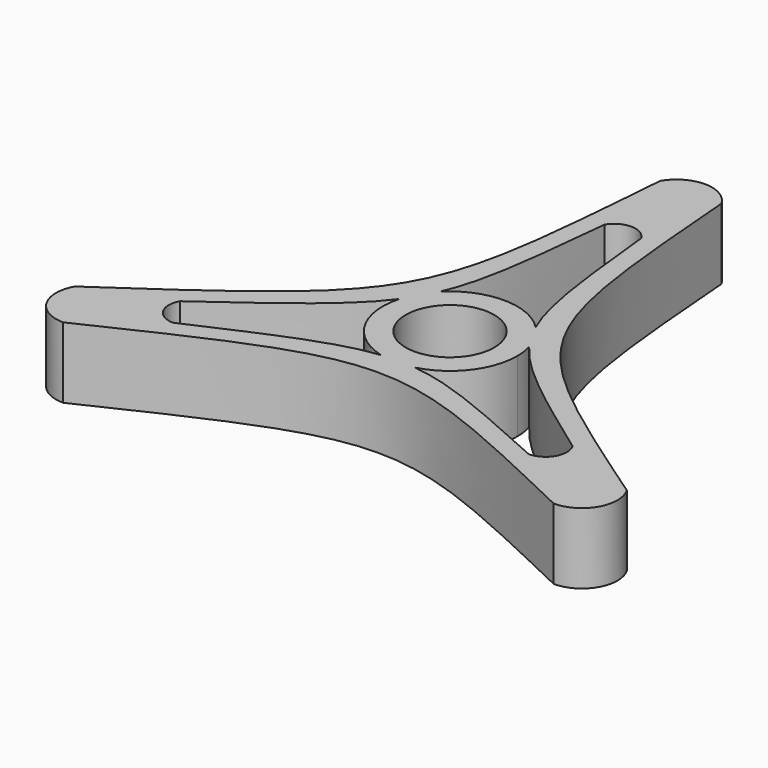
from build123d import *

# Parameters (mm, degrees)
F0_R     = 6.25
F1_DEPTH = 10


# Not quite as in the source:
# - a feature names something its author has since deleted; it is built from what else it names


with BuildPart() as f1:
    # F0 (on Top) → F1 (new body)
    with BuildSketch(Plane.XY):
        with BuildLine():
            add(Edge.make_bspline(
                [(4.3301272175, 42.4999999798), (7.3612159322, 4.25), (7.3612159322, 4.25), (38.9711430885, -17.5000001821)],
                knots=[0, 0, 0, 0, 69.2820323028, 69.2820323028, 69.2820323028, 69.2820323028], degree=3))
            ThreePointArc((4.3301272175, 42.4999999798), (2.102e-07, 45), (-4.3301268204, 42.5000000202))
            add(Edge.make_bspline(
                [(-38.9711432521, -17.4999998179), (-7.3612159322, 4.25), (-7.3612159322, 4.25), (-4.3301268204, 42.5000000202)],
                knots=[0, 0, 0, 0, 69.2820323028, 69.2820323028, 69.2820323028, 69.2820323028], degree=3))
            ThreePointArc((-38.9711432521, -17.4999998179), (-38.9711432754, -22.4999998179), (-34.6410162682, -24.9999998382))
            add(Edge.make_bspline(
                [(-34.6410162682, -24.9999998382), (0, -8.5), (0, -8.5), (34.6410160346, -25.0000001618)],
                knots=[0, 0, 0, 0, 69.2820323028, 69.2820323028, 69.2820323028, 69.2820323028], degree=3))
            ThreePointArc((34.6410160346, -25.0000001618), (38.9711430652, -22.5000001821), (38.9711430885, -17.5000001821))
        make_face()
        with BuildLine():
            ThreePointArc((6.7724364928, 6.6621395926), (8.2272413629, 4.7499999534), (9.1558004059, 2.5340321482))
            add(Edge.make_bspline(
                [(9.1558004059, 2.5340321482), (12.4794508791, -1.9849209314), (17.9661663578, -5.9523055453), (27.7128128343, -13.0000001849)],
                knots=[28.2758618531, 28.2758618531, 28.2758618531, 28.2758618531, 50.2294734195, 50.2294734195, 50.2294734195, 50.2294734195], degree=3))
            ThreePointArc((27.7128128343, -13.0000001849), (27.7128128143, -16.0000001849), (25.114736593, -17.5000001676))
            add(Edge.make_bspline(
                [(25.114736593, -17.5000001676), (14.1379308325, -12.5830038779), (7.9587172847, -9.8150611129), (2.3833638843, -9.1961718446)],
                knots=[0, 0, 0, 0, 21.953611623, 21.953611623, 21.953611623, 21.953611623], degree=3))
            ThreePointArc((2.3833638843, -9.1961718446), (-5.39e-08, -9.5), (-2.3833639886, -9.1961718175))
            add(Edge.make_bspline(
                [(-2.3833639886, -9.1961718175), (-7.9587173906, -9.8150610209), (-14.1379309923, -12.5830037018), (-25.1147368265, -17.4999998324)],
                knots=[28.2758618531, 28.2758618531, 28.2758618531, 28.2758618531, 50.2294734195, 50.2294734195, 50.2294734195, 50.2294734195], degree=3))
            ThreePointArc((-25.1147368265, -17.4999998324), (-27.7128130279, -15.9999998151), (-27.7128130079, -12.9999998151))
            add(Edge.make_bspline(
                [(-9.1558003771, 2.534032252), (-12.4794509058, -1.9849207937), (-17.9661664304, -5.9523053189), (-27.7128130079, -12.9999998151)],
                knots=[28.2758617965, 28.2758617965, 28.2758617965, 28.2758617965, 50.2294734195, 50.2294734195, 50.2294734195, 50.2294734195], degree=3))
            ThreePointArc((-9.1558003771, 2.534032252), (-8.227241309, 4.7500000466), (-6.7724364173, 6.6621396694))
            add(Edge.make_bspline(
                [(-2.5980760078, 30.5000000173), (-3.8282353656, 18.5353092472), (-4.5207334885, 11.7999819523), (-6.7724364173, 6.6621396694)],
                knots=[0, 0, 0, 0, 21.9536115664, 21.9536115664, 21.9536115664, 21.9536115664], degree=3))
            ThreePointArc((-2.5980760078, 30.5000000173), (2.136e-07, 32), (2.5980764149, 30.4999999827))
            add(Edge.make_bspline(
                [(2.5980764149, 30.4999999827), (3.8282355979, 18.5353091968), (4.5207336211, 11.7999819066), (6.7724364928, 6.6621395926)],
                knots=[0, 0, 0, 0, 21.953611623, 21.953611623, 21.953611623, 21.953611623], degree=3))
        make_face(mode=Mode.SUBTRACT)
        with BuildLine():
            add(Edge.make_bspline(
                [(6.7724364928, 6.6621395926), (7.4208869274, 5.1825322592), (8.1986480984, 3.8354103774), (9.1558004059, 2.5340321482)],
                knots=[21.953611623, 21.953611623, 21.953611623, 21.953611623, 28.2758618531, 28.2758618531, 28.2758618531, 28.2758618531], degree=3))
            ThreePointArc((9.1558004059, 2.5340321482), (8.2272413629, 4.7499999534), (6.7724364928, 6.6621395926))
        make_face()
        with BuildLine():
            ThreePointArc((-2.3833639886, -9.1961718175), (-5.39e-08, -9.5), (2.3833638843, -9.1961718446))
            add(Edge.make_bspline(
                [(2.3833638843, -9.1961718446), (0.7777611287, -9.0179427274), (-0.7777612284, -9.0179427186), (-2.3833639886, -9.1961718175)],
                knots=[21.953611623, 21.953611623, 21.953611623, 21.953611623, 28.2758618531, 28.2758618531, 28.2758618531, 28.2758618531], degree=3))
        make_face()
        with BuildLine():
            add(Edge.make_bspline(
                [(-6.7724364173, 6.6621396694), (-7.42088687, 5.1825323411), (-8.1986480561, 3.8354104682), (-9.1558003771, 2.534032252)],
                knots=[21.9536115664, 21.9536115664, 21.9536115664, 21.9536115664, 28.2758617965, 28.2758617965, 28.2758617965, 28.2758617965], degree=3))
            ThreePointArc((-6.7724364173, 6.6621396694), (-8.227241309, 4.7500000466), (-9.1558003771, 2.534032252))
        make_face()
        with BuildLine():
            ThreePointArc((2.3833638843, -9.1961718446), (7.5130538698, -5.814122595), (9.5, 0))
            ThreePointArc((9.5, 0), (9.413556816, 1.2786508797), (9.1558004059, 2.5340321482))
            add(Edge.make_bspline(
                [(6.7724364928, 6.6621395926), (7.4208869274, 5.1825322592), (8.1986480984, 3.8354103774), (9.1558004059, 2.5340321482)],
                knots=[21.953611623, 21.953611623, 21.953611623, 21.953611623, 28.2758618531, 28.2758618531, 28.2758618531, 28.2758618531], degree=3))
            ThreePointArc((6.7724364928, 6.6621395926), (5.39e-08, 9.5), (-6.7724364173, 6.6621396694))
            add(Edge.make_bspline(
                [(-6.7724364173, 6.6621396694), (-7.42088687, 5.1825323411), (-8.1986480561, 3.8354104682), (-9.1558003771, 2.534032252)],
                knots=[21.9536115664, 21.9536115664, 21.9536115664, 21.9536115664, 28.2758617965, 28.2758617965, 28.2758617965, 28.2758617965], degree=3))
            ThreePointArc((-9.1558003771, 2.534032252), (-8.2272413629, -4.7499999534), (-2.3833639886, -9.1961718175))
            add(Edge.make_bspline(
                [(2.3833638843, -9.1961718446), (0.7777611287, -9.0179427274), (-0.7777612284, -9.0179427186), (-2.3833639886, -9.1961718175)],
                knots=[21.953611623, 21.953611623, 21.953611623, 21.953611623, 28.2758618531, 28.2758618531, 28.2758618531, 28.2758618531], degree=3))
        make_face()
        Circle(F0_R, mode=Mode.SUBTRACT)
    extrude(amount=F1_DEPTH)


solid = f1.part
